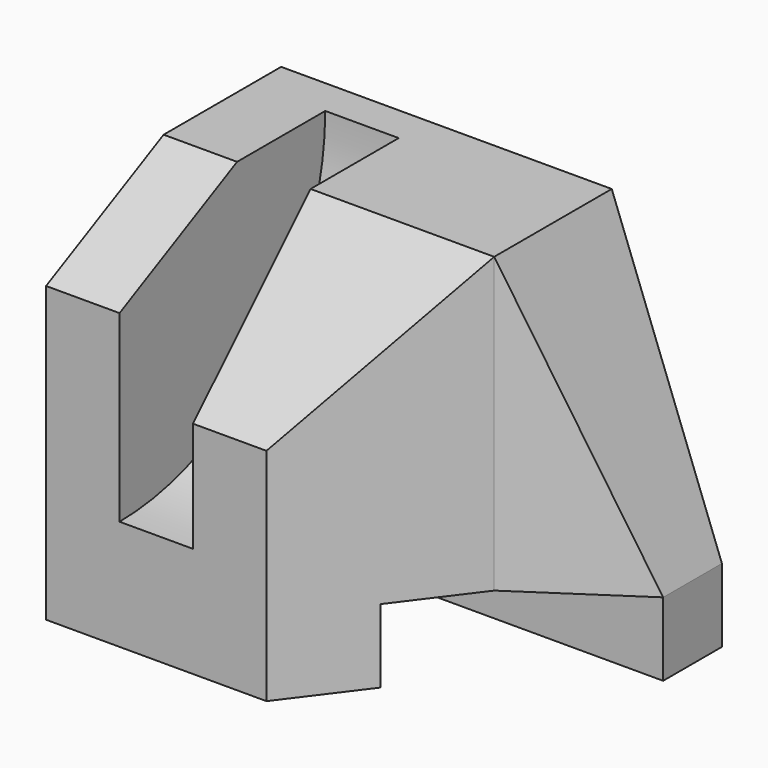
from build123d import *

# Parameters (mm, degrees)
F0_W      = 60
F0_H      = 40
F1_DEPTH  = 50
F3_W      = 10
F3_H      = 35
F5_DEPTH  = 35
F6_R      = 34.99999
F7_DEPTH  = 12.7
F9_DEPTH  = 40
F10_DEPTH = 50.001
F12_DEPTH = 20.001
F13_W     = 20
F13_H     = 10
F14_DEPTH = 60.001


# Not quite as in the source:
# - a fillet or chamfer is up to 0.001 mm smaller than in the source, because OpenCascade refuses the exact size


with BuildPart() as f1:
    # F0 (on Top) → F1 (new body)
    with BuildSketch(Plane.XY):
        with Locations((30, -20)):
            Rectangle(F0_W, F0_H)
    extrude(amount=F1_DEPTH)

    # F3 (on face) → F5 (cut, through all)
    with BuildSketch(Plane.XY.offset(50)):
        with Locations((15, -22.5)):
            Rectangle(F3_W, F3_H)
    extrude(amount=-F5_DEPTH, mode=Mode.SUBTRACT)

    # F6 (radius 35 in the source; OpenCascade refuses exactly that, so slightly less here)
    f6_edges = [f1.edges().sort_by_distance(p)[0] for p in [
        (15, -5, 15),
    ]]
    fillet(f6_edges, radius=F6_R)

    # F2 (on face) → F7 (cut)
    with BuildSketch(Plane(origin=(0, 0, 0), x_dir=(0, -1, 0), z_dir=(-1, 0, 0))):
        Polygon((40, 50), (20, 50), (40, 40), align=None)
    extrude(amount=-F7_DEPTH, mode=Mode.SUBTRACT)

    # F8 (on face) → F9 (cut, through all)
    with BuildSketch(Plane.YZ.offset(60)):
        Polygon((-40, 30), (-20, 50), (-40, 50), align=None)
    extrude(amount=-F9_DEPTH, mode=Mode.SUBTRACT)

    # F3 (on face) → F10 (cut, through all)
    with BuildSketch(Plane.XY.offset(50)):
        Polygon((45, -20), (30, -40), (60, -40), (60, -10), align=None)
    extrude(amount=-F10_DEPTH, mode=Mode.SUBTRACT)

    # F11 (on face) → F12 (cut, through all)
    with BuildSketch(Plane(origin=(0, 0, 0), x_dir=(-1, 0, 0), z_dir=(0, 1, 0))):
        Polygon((-60, 10), (-45, 50), (-60, 50), align=None)
    extrude(amount=-F12_DEPTH, mode=Mode.SUBTRACT)

    # F13 (on face) → F14 (cut, through all)
    with BuildSketch(Plane(origin=(0, 0, 0), x_dir=(0, -1, 0), z_dir=(-1, 0, 0))):
        with Locations((20, 5)):
            Rectangle(F13_W, F13_H)
    extrude(amount=-F14_DEPTH, mode=Mode.SUBTRACT)


solid = f1.part
